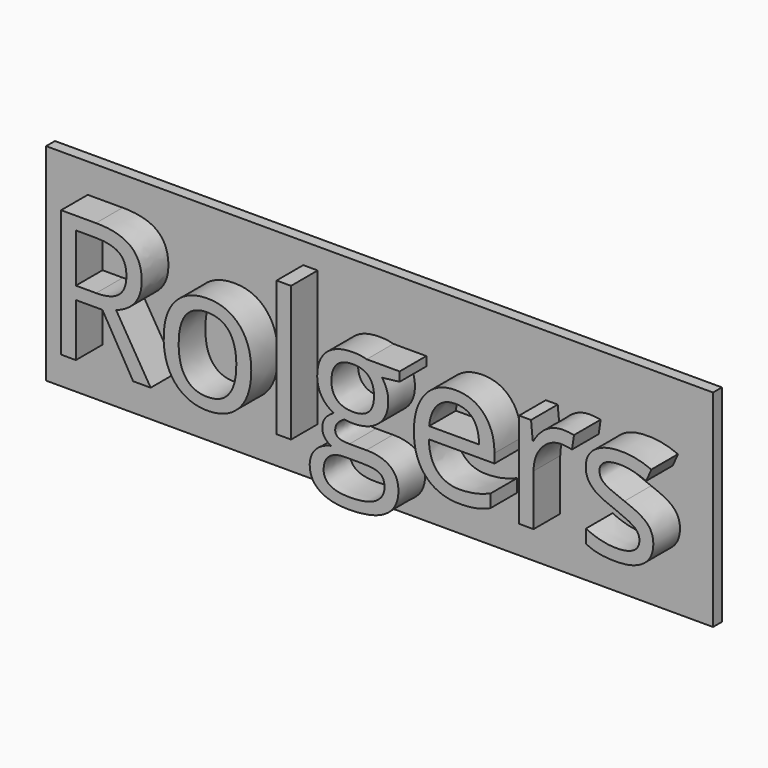
from build123d import *

# Parameters (mm, degrees)
F0_W         = 152.4614542723
F0_H         = 47.1948389895
F1_DEPTH     = 2.54
F2_TEXT_SIZE = 40.7116933881
F3_DEPTH     = 7.62


# Not quite as in the source:
# - Text() gives the source's letters only with a copy of the font that has no kerning and outlines rounded to 1/6400 em; it was checked with that copy


with BuildPart() as f1:
    # F0 (on Front) → F1 (new body)
    with BuildSketch(Plane.XZ):
        with Locations((-0.0153630972, 15.9466934856)):
            Rectangle(F0_W, F0_H)
    extrude(amount=F1_DEPTH)

    # F2 (on face) → F3 (join)
    with BuildSketch(Plane.XZ.offset(2.54)):
        with Locations((-70.7154497504, 3.7792748772)):
            Text('Rolgers', F2_TEXT_SIZE, font='Open Sans', text_align=(TextAlign.LEFT, TextAlign.BOTTOM))
    extrude(amount=F3_DEPTH)


solid = f1.part
